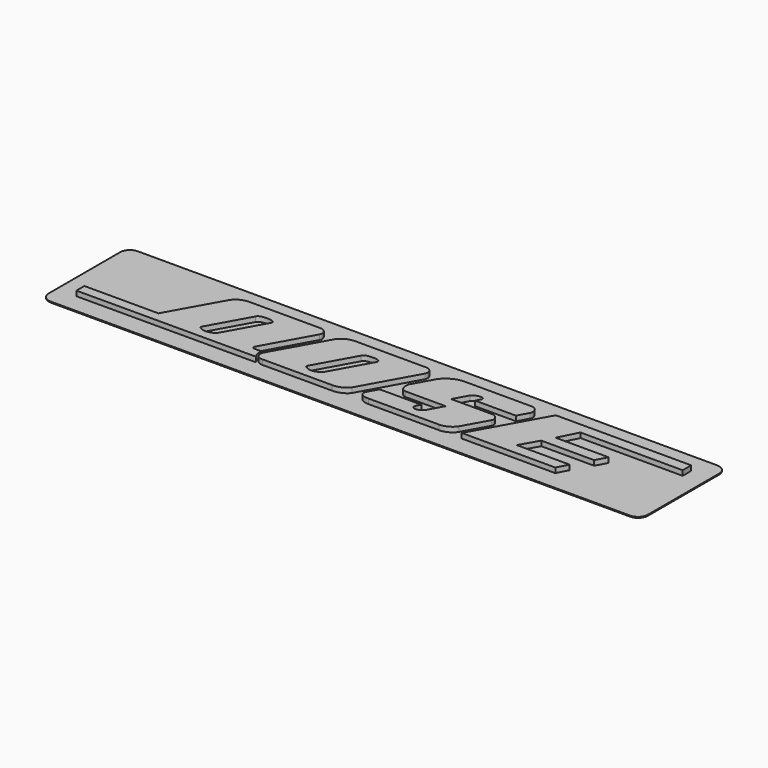
from build123d import *

# Parameters (mm, degrees)
F1_DEPTH = 5
F2_W     = 604.2038831239
F2_H     = 109.7505224343
F3_DEPTH = 1
F4_R     = 10


# Not quite as in the source:
# - ends of sketch curves that miss each other by under 0.0002 mm in the source are joined


with BuildPart() as f1:
    # F0 (on Top) → F1 (new body)
    with BuildSketch(Plane.XY):
        with BuildLine():
            add(Edge.make_bspline(
                [(82.5151938945, 91.4469261483), (84.2045618945, 94.7999181483), (81.5236258945, 101.2010621483), (76.6392178945, 100.8962381483)],
                knots=[0, 0, 0, 0, 1, 1, 1, 1], degree=3))
            add(Edge.make_bspline(
                [(76.6392178945, 100.8962381483), (74.3622738945, 100.8962381483), (10.4977698945, 100.8962381483), (8.3677298945, 100.8962381483)],
                knots=[0, 0, 0, 0, 1, 1, 1, 1], degree=3))
            add(Edge.make_bspline(
                [(8.3677298945, 100.8962381483), (0.7656978945, 100.8962381483), (-8.1584621055, 95.7914941483), (-11.4269741055, 89.6180461483)],
                knots=[0, 0, 0, 0, 1, 1, 1, 1], degree=3))
            add(Edge.make_bspline(
                [(-11.4269741055, 89.6180461483), (-12.1981741055, 87.9433901483), (-21.0488621055, 72.2435261483), (-22.1139021055, 70.4146141483)],
                knots=[0, 0, 0, 0, 1, 1, 1, 1], degree=3))
            add(Edge.make_bspline(
                [(-22.1139021055, 70.4146141483), (-24.0970381055, 66.9110461483), (-22.4811421055, 58.6038941483), (-16.9356861055, 58.8315901483)],
                knots=[0, 0, 0, 0, 1, 1, 1, 1], degree=3))
            Line((-16.9356861055, 58.8315901483), (23.3147378945, 58.8315901483))
            Line((23.3147378945, 58.8315901483), (15.5290818945, 44.7366061483))
            add(Edge.make_bspline(
                [(15.5290818945, 44.7366061483), (12.3340098945, 38.7908461483), (2.2714098945, 38.4088941483), (4.5483538945, 44.6594701483)],
                knots=[0, 0, 0, 0, 1, 1, 1, 1], degree=3))
            Line((4.5483538945, 44.6594701483), (6.8620178945, 48.8497821483))
            Line((6.8620178945, 48.8497821483), (-35.2981101055, 48.7726541483))
            Line((-35.2981101055, 48.7726541483), (-40.9170301055, 38.4088941483))
            add(Edge.make_bspline(
                [(-40.9170301055, 38.4088941483), (-43.3041341055, 33.9908941483), (-37.9423261055, 30.7884861483), (-32.2499661055, 31.0933101483)],
                knots=[0, 0, 0, 0, 1, 1, 1, 1], degree=3))
            add(Edge.make_bspline(
                [(-32.2499661055, 31.0933101483), (-31.6990701055, 31.0933101483), (36.6458498945, 31.0933101483), (38.7758898945, 31.0933101483)],
                knots=[0, 0, 0, 0, 1, 1, 1, 1], degree=3))
            add(Edge.make_bspline(
                [(38.7758898945, 31.0933101483), (44.6518738945, 31.0198781483), (50.4544178945, 34.3728461483), (52.9516978945, 38.6402861483)],
                knots=[0, 0, 0, 0, 1, 1, 1, 1], degree=3))
            add(Edge.make_bspline(
                [(52.9516978945, 38.6402861483), (53.1720418945, 39.0185421483), (65.9890098945, 61.8797661483), (66.3562818945, 62.6436381483)],
                knots=[0, 0, 0, 0, 1, 1, 1, 1], degree=3))
            add(Edge.make_bspline(
                [(66.3562818945, 62.6436381483), (68.1190498945, 66.6062541483), (64.9974338945, 71.0242621483), (60.1864898945, 71.0242621483)],
                knots=[0, 0, 0, 0, 1, 1, 1, 1], degree=3))
            Line((60.1864898945, 71.0242621483), (19.0546578945, 71.0242621483))
            Line((19.0546578945, 71.0242621483), (26.9504898945, 85.2000381483))
            add(Edge.make_bspline(
                [(26.9504898945, 85.2000381483), (29.4110578945, 88.5530061483), (39.2533138945, 90.5324861483), (38.2250338945, 85.6554301483)],
                knots=[0, 0, 0, 0, 1, 1, 1, 1], degree=3))
            Line((38.2250338945, 85.6554301483), (35.4339458945, 80.7783741483))
            Line((35.4339458945, 80.7783741483), (76.5657778945, 80.7783741483))
            Line((76.5657778945, 80.7783741483), (82.5151938945, 91.4469261483))
        make_face()
    extrude(amount=F1_DEPTH)


with BuildPart() as f1b:
    # F0 (on Top) → F1, piece 2 (new body)
    with BuildSketch(Plane.XY):
        Polygon((237.2737218945, 100.8962381483), (100.7307218945, 100.8962381483), (61.7289218945, 31.0933101483), (156.0383618945, 31.0933101483), (161.7674418945, 41.9932541483), (108.5164018945, 41.9932541483), (118.7993698945, 60.0508541483), (172.1238498945, 60.0508541483), (177.9263618945, 70.9507901483), (124.4916978945, 70.9507901483), (134.1870578945, 90.1542221483), (237.2737218945, 90.1542221483), align=None)
    extrude(amount=F1_DEPTH)


with BuildPart() as f1c:
    # F0 (on Top) → F1, piece 3 (new body)
    with BuildSketch(Plane.XY):
        with BuildLine():
            add(Edge.make_bspline(
                [(-24.0970381055, 92.1337021483), (-22.1139021055, 96.0963181483), (-25.3824141055, 101.1275981483), (-30.1199261055, 100.8962381483)],
                knots=[0, 0, 0, 0, 1, 1, 1, 1], degree=3))
            add(Edge.make_bspline(
                [(-30.1199261055, 100.8962381483), (-32.3233981055, 100.8962381483), (-98.8321181055, 100.8962381483), (-100.2276461055, 100.8962381483)],
                knots=[0, 0, 0, 0, 1, 1, 1, 1], degree=3))
            add(Edge.make_bspline(
                [(-100.2276461055, 100.8962381483), (-107.4624701055, 101.2010621483), (-113.3384141055, 98.3842461483), (-116.6803981055, 92.6661901483)],
                knots=[0, 0, 0, 0, 1, 1, 1, 1], degree=3))
            add(Edge.make_bspline(
                [(-116.6803981055, 92.6661901483), (-117.7454061055, 90.8373101483), (-144.8850861055, 42.2980781483), (-145.4726621055, 41.1522461483)],
                knots=[0, 0, 0, 0, 1, 1, 1, 1], degree=3))
            add(Edge.make_bspline(
                [(-145.4726621055, 41.1522461483), (-147.7128861055, 37.4944541483), (-146.0969901055, 30.7884861483), (-139.0825341055, 31.0933101483)],
                knots=[0, 0, 0, 0, 1, 1, 1, 1], degree=3))
            add(Edge.make_bspline(
                [(-139.0825341055, 31.0933101483), (-135.1897261055, 31.0933101483), (-71.6557181055, 31.0198781483), (-69.1951501055, 31.0933101483)],
                knots=[0, 0, 0, 0, 1, 1, 1, 1], degree=3))
            add(Edge.make_bspline(
                [(-69.1951501055, 31.0933101483), (-62.5112221055, 30.9427501483), (-56.7087101055, 34.2185821483), (-54.2481421055, 37.8764061483)],
                knots=[0, 0, 0, 0, 1, 1, 1, 1], degree=3))
            add(Edge.make_bspline(
                [(-54.2481421055, 37.8764061483), (-53.2198541055, 39.4775981483), (-25.0886061055, 90.3819181483), (-24.0970381055, 92.1337021483)],
                knots=[0, 0, 0, 0, 1, 1, 1, 1], degree=3))
        make_face()
        with BuildLine():
            add(Edge.make_bspline(
                [(-82.5997341055, 84.5132941483), (-83.5178381055, 82.9892061483), (-104.0470541055, 45.9558701483), (-104.8549981055, 44.4317821483)],
                knots=[0, 0, 0, 0, 1, 1, 1, 1], degree=3))
            add(Edge.make_bspline(
                [(-71.8026221055, 87.8662621483), (-73.6388541055, 87.8662621483), (-81.2409181055, 88.0939581483), (-82.5997341055, 84.5132941483)],
                knots=[0, 0, 0, 0, 1, 1, 1, 1], degree=3))
            add(Edge.make_bspline(
                [(-66.0735421055, 83.9036461483), (-64.7147341055, 86.6469981483), (-69.6725821055, 87.8662621483), (-71.8026221055, 87.8662621483)],
                knots=[0, 0, 0, 0, 1, 1, 1, 1], degree=3))
            add(Edge.make_bspline(
                [(-88.0350061055, 44.4317821483), (-86.6394781055, 46.7160781483), (-66.9916781055, 82.3795581483), (-66.0735421055, 83.9036461483)],
                knots=[0, 0, 0, 0, 1, 1, 1, 1], degree=3))
            add(Edge.make_bspline(
                [(-98.0976061055, 40.2378061483), (-96.3348301055, 40.2378061483), (-90.2384861055, 41.0788141483), (-88.0350061055, 44.4317821483)],
                knots=[0, 0, 0, 0, 1, 1, 1, 1], degree=3))
            add(Edge.make_bspline(
                [(-104.8549981055, 44.4317821483), (-105.6996701055, 42.0666861483), (-100.2276461055, 40.2378061483), (-98.0976061055, 40.2378061483)],
                knots=[0, 0, 0, 0, 1, 1, 1, 1], degree=3))
        make_face(mode=Mode.SUBTRACT)
    extrude(amount=F1_DEPTH)


with BuildPart() as f1d:
    # F0 (on Top) → F1, piece 4 (new body)
    with BuildSketch(Plane.XY):
        with BuildLine():
            Line((-252.2318301055, 41.1522461483), (-326.9301591055, 41.1522461483))
            Line((-326.9301591055, 41.1522461483), (-326.9301612294, 31.0933121764))
            Line((-326.9301612294, 31.0933121764), (-145.8930078568, 31.4100798102))
            Line((-145.8930078568, 31.4100798102), (-146.3136309451, 31.8951456212))
            add(Edge.make_bspline(
                [(-147.7078150367, 41.169564047), (-147.8400716725, 40.8603092989), (-148.1956924991, 39.8641003291), (-148.4874092275, 38.0980773888), (-148.3385490278, 35.8969158924), (-147.6592558078, 33.7662872867), (-146.8235608029, 32.4725168869), (-146.3136309451, 31.8951456212)],
                knots=[0.0666780463, 0.0666780463, 0.0666780463, 0.0666780463, 0.125, 0.25, 0.375, 0.5, 0.6211481623, 0.6211481623, 0.6211481623, 0.6211481623], degree=3))
            Line((-147.7078150367, 41.169564047), (-155.7288993945, 41.274537809))
            ThreePointArc((-155.7288993945, 41.274537809), (-157.4339768829, 42.2730002596), (-157.4492495905, 44.2488502669))
            add(Edge.make_bspline(
                [(-157.4492495905, 44.2488502669), (-149.6836228827, 58.1669170435), (-131.5368302166, 90.9972645978), (-130.7439299006, 92.3980662445)],
                knots=[0.200357095, 0.200357095, 0.200357095, 0.200357095, 1, 1, 1, 1], degree=3))
            add(Edge.make_bspline(
                [(-130.7439299006, 92.3980662445), (-128.7607939006, 96.3606822445), (-132.0293059006, 101.3919622445), (-136.7668179006, 101.1606022445)],
                knots=[0, 0, 0, 0, 1, 1, 1, 1], degree=3))
            add(Edge.make_bspline(
                [(-136.7668179006, 101.1606022445), (-138.9702899006, 101.1606022445), (-205.4790099006, 101.1606022445), (-206.8745379006, 101.1606022445)],
                knots=[0, 0, 0, 0, 1, 1, 1, 1], degree=3))
            add(Edge.make_bspline(
                [(-206.8745379006, 101.1606022445), (-214.1093619006, 101.4654262445), (-219.9853059006, 98.6486102445), (-223.3272899006, 92.9305542445)],
                knots=[0, 0, 0, 0, 1, 1, 1, 1], degree=3))
            add(Edge.make_bspline(
                [(-223.3272899006, 92.9305542445), (-224.3922979006, 91.1016742445), (-251.5319779006, 42.5624422445), (-252.1195539006, 41.4166102445)],
                knots=[0, 0, 0, 0, 1, 1, 1, 1], degree=3))
            Line((-252.1195539006, 41.4166102445), (-252.2318301055, 41.1522461483))
        make_face()
        with BuildLine():
            add(Edge.make_bspline(
                [(-189.2466259006, 84.7776582445), (-190.1647299006, 83.2535702445), (-210.6939459006, 46.2202342445), (-211.5018899006, 44.6961462445)],
                knots=[0, 0, 0, 0, 1, 1, 1, 1], degree=3))
            add(Edge.make_bspline(
                [(-178.4495139006, 88.1306262445), (-180.2857459006, 88.1306262445), (-187.8878099006, 88.3583222445), (-189.2466259006, 84.7776582445)],
                knots=[0, 0, 0, 0, 1, 1, 1, 1], degree=3))
            add(Edge.make_bspline(
                [(-172.7204339006, 84.1680102445), (-171.3616259006, 86.9113622445), (-176.3194739006, 88.1306262445), (-178.4495139006, 88.1306262445)],
                knots=[0, 0, 0, 0, 1, 1, 1, 1], degree=3))
            add(Edge.make_bspline(
                [(-194.6818979006, 44.6961462445), (-193.2863699006, 46.9804422445), (-173.6385699006, 82.6439222445), (-172.7204339006, 84.1680102445)],
                knots=[0, 0, 0, 0, 1, 1, 1, 1], degree=3))
            add(Edge.make_bspline(
                [(-204.7444979006, 40.5021702445), (-202.9817219006, 40.5021702445), (-196.8853779006, 41.3431782445), (-194.6818979006, 44.6961462445)],
                knots=[0, 0, 0, 0, 1, 1, 1, 1], degree=3))
            add(Edge.make_bspline(
                [(-211.5018899006, 44.6961462445), (-212.3465619006, 42.3310502445), (-206.8745379006, 40.5021702445), (-204.7444979006, 40.5021702445)],
                knots=[0, 0, 0, 0, 1, 1, 1, 1], degree=3))
        make_face(mode=Mode.SUBTRACT)
    extrude(amount=F1_DEPTH)


with BuildPart() as f3:
    # F2 (on face) → F3 (new body)
    with BuildSketch(Plane(origin=(0, 0, 0), x_dir=(1, 0, 0), z_dir=(0, 0, -1))):
        with Locations((-44.8282196674, -66.2853410274)):
            Rectangle(F2_W, F2_H)
    extrude(amount=F3_DEPTH)

    # F4
    f4_edges = [f3.edges().sort_by_distance(p)[0] for p in [
        (-346.930161, 121.160602, -0.5),
        (-346.930161, 11.41008, -0.5),
        (257.273722, 11.41008, -0.5),
        (257.273722, 121.160602, -0.5),
    ]]
    fillet(f4_edges, radius=F4_R)


solid = Compound([f1.part, f1b.part, f1c.part, f1d.part, f3.part])
